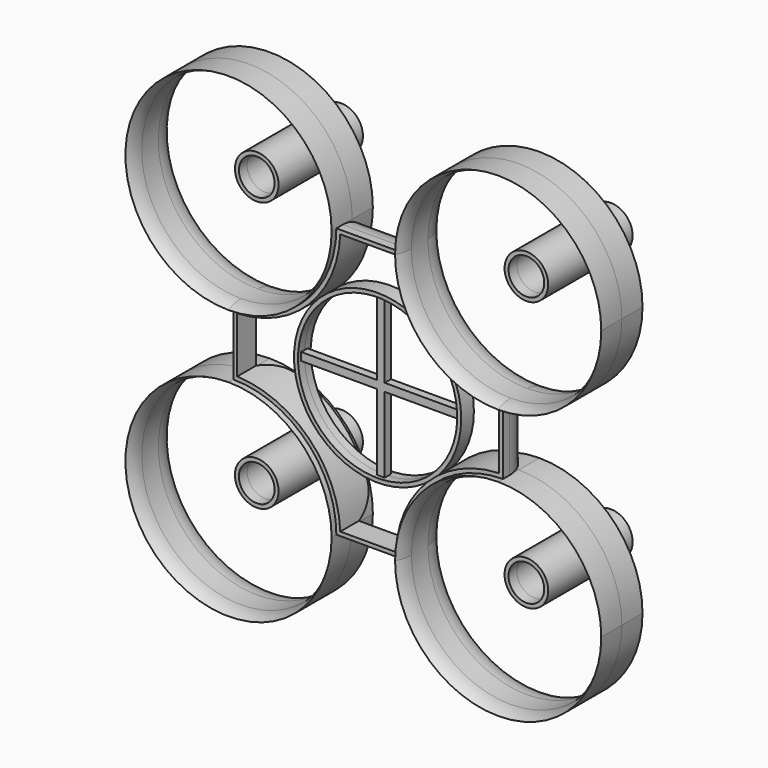
from build123d import *

# Parameters (mm, degrees)
F1_DEPTH       = 4.1275
F2_DEPTH       = 3.175
F3_R           = 15.875
F4_DEPTH       = 25.4
F6_DEPTH       = 25.4
F7_T2_ANGLE    = 270
F7_T4_ANGLE    = 90
F7_T6_ANGLE    = 270
F7_T8_ANGLE    = 90
F7_2_T2_ANGLE  = 90
F7_2_T4_ANGLE  = 270
F7_2_T6_ANGLE  = 90
F7_2_T8_ANGLE  = 270
F7_3_T2_ANGLE  = 90
F7_3_T4_ANGLE  = 89.999999553
F7_3_T6_ANGLE  = 180.000000447
F7_3_T8_ANGLE  = 90
F7_3_T10_ANGLE = 89.999999553
F7_3_T12_ANGLE = 180.000000447
F7_4_T2_ANGLE  = 180
F7_4_T4_ANGLE  = 89.999999553
F7_4_T6_ANGLE  = 90.000000447
F7_4_T8_ANGLE  = 180
F7_4_T10_ANGLE = 89.999999553
F7_4_T12_ANGLE = 90.000000447
F8_T1_DEPTH    = 35.56
F8_T3_DEPTH    = 35.56
F9_R           = 13.3878708116
F10_DEPTH      = 1.27
F11_DEPTH      = 0.635
F12_R          = 3.4925
F12_R_2        = 2.8575
F13_DEPTH      = 15.24
F13_DEPTH_BACK = 1.651


# Not quite as in the source:
# - a fillet or chamfer that OpenCascade refuses, or shapes differently, is made with other operations: its cross-section is extruded or revolved along the edge and cut away or added


with BuildPart() as f1:
    # F0 (on Front) → F1 (new body, symmetric)
    with BuildSketch(Plane.XZ):
        with BuildLine():
            ThreePointArc((-21.59, 5.08), (-9.9156670426, 9.9156670426), (-5.08, 21.59))
            ThreePointArc((-5.08, 21.59), (-33.2643329574, 33.2643329574), (-21.59, 5.08))
        make_face()
    extrude(amount=F1_DEPTH, both=True)


with BuildPart() as f1b:
    # F0 (on Front) → F1, piece 2 (new body, symmetric)
    with BuildSketch(Plane.XZ):
        with BuildLine():
            ThreePointArc((-5.08, -21.59), (-9.9156670426, -9.9156670426), (-21.59, -5.08))
            ThreePointArc((-21.59, -5.08), (-33.2643329574, -33.2643329574), (-5.08, -21.59))
        make_face()
    extrude(amount=F1_DEPTH, both=True)


with BuildPart() as f1c:
    # F0 (on Front) → F1, piece 3 (new body, symmetric)
    with BuildSketch(Plane.XZ):
        with BuildLine():
            ThreePointArc((38.1, -21.59), (33.2643329574, -9.9156670426), (21.59, -5.08))
            ThreePointArc((21.59, -5.08), (9.9156670426, -9.9156670426), (5.08, -21.59))
            ThreePointArc((5.08, -21.59), (21.59, -38.1), (38.1, -21.59))
        make_face()
    extrude(amount=F1_DEPTH, both=True)


with BuildPart() as f1d:
    # F0 (on Front) → F1, piece 4 (new body, symmetric)
    with BuildSketch(Plane.XZ):
        with BuildLine():
            ThreePointArc((38.1, 21.59), (21.59, 38.1), (5.08, 21.59))
            ThreePointArc((5.08, 21.59), (9.9156670426, 9.9156670426), (21.59, 5.08))
            ThreePointArc((21.59, 5.08), (33.2643329574, 9.9156670426), (38.1, 21.59))
        make_face()
    extrude(amount=F1_DEPTH, both=True)


with BuildPart() as f2:
    # F0 (on Front) → F2 (new body, symmetric)
    with BuildSketch(Plane.XZ):
        with BuildLine():
            Line((5.08, 21.59), (-5.08, 21.59))
            ThreePointArc((-5.08, 21.59), (-9.9156670426, 9.9156670426), (-21.59, 5.08))
            Line((-21.59, 5.08), (-21.59, -5.08))
            ThreePointArc((-21.59, -5.08), (-9.9156670426, -9.9156670426), (-5.08, -21.59))
            Line((-5.08, -21.59), (5.08, -21.59))
            ThreePointArc((5.08, -21.59), (9.9156670426, -9.9156670426), (21.59, -5.08))
            Line((21.59, -5.08), (21.59, 5.08))
            ThreePointArc((21.59, 5.08), (9.9156670426, 9.9156670426), (5.08, 21.59))
        make_face()
    extrude(amount=F2_DEPTH, both=True)

    # F5 (on face) → F6 (cut)
    with BuildSketch(Plane.XZ.offset(3.175)):
        with BuildLine():
            ThreePointArc((20.955, 4.4567632947), (9.4666542366, 9.4666542366), (4.4567632947, 20.955))
            Line((4.4567632947, 20.955), (-4.4567632947, 20.955))
            ThreePointArc((-4.4567632947, 20.955), (-9.4666542366, 9.4666542366), (-20.955, 4.4567632947))
            Line((-20.955, 4.4567632947), (-20.955, -4.4567632947))
            ThreePointArc((-20.955, -4.4567632947), (-9.4666542366, -9.4666542366), (-4.4567632947, -20.955))
            Line((-4.4567632947, -20.955), (4.4567632947, -20.955))
            ThreePointArc((4.4567632947, -20.955), (9.4666542366, -9.4666542366), (20.955, -4.4567632947))
            Line((20.955, -4.4567632947), (20.955, 4.4567632947))
        make_face()
    extrude(amount=-F6_DEPTH, mode=Mode.SUBTRACT)

    # F8: fillet of radius 5.08 on 4 edges, made by hand

    # F8_s2 → F8_t1 (cut)
    with BuildSketch(Plane.YZ.offset(-17.78)):
        with BuildLine():
            ThreePointArc((3.175, 16.51), (1.6871024484, 20.1021024484), (-1.905, 21.59))
            Line((-1.905, 21.59), (3.175, 21.59))
            Line((3.175, 21.59), (3.175, 16.51))
        make_face()
        with BuildLine():
            ThreePointArc((3.175, -16.51), (1.6871024484, -20.1021024484), (-1.905, -21.59))
            Line((-1.905, -21.59), (3.175, -21.59))
            Line((3.175, -21.59), (3.175, -16.51))
        make_face()
    extrude(amount=F8_T1_DEPTH, mode=Mode.SUBTRACT)

    # F8_s4 → F8_t3 (cut)
    with BuildSketch(Plane.XY.offset(-17.78)):
        with BuildLine():
            ThreePointArc((16.51, 3.175), (20.1021024484, 1.6871024484), (21.59, -1.905))
            Line((21.59, -1.905), (21.59, 3.175))
            Line((21.59, 3.175), (16.51, 3.175))
        make_face()
        with BuildLine():
            ThreePointArc((-16.51, 3.175), (-20.1021024484, 1.6871024484), (-21.59, -1.905))
            Line((-21.59, -1.905), (-21.59, 3.175))
            Line((-21.59, 3.175), (-16.51, 3.175))
        make_face()
    extrude(amount=F8_T3_DEPTH, mode=Mode.SUBTRACT)


with BuildPart() as f4_tool:
    # F3 (on face) → F4 (new body)
    with BuildSketch(Plane.XZ.offset(4.1275)):
        with Locations((-21.59, 21.59)):
            Circle(F3_R)
        with Locations((21.59, 21.59)):
            Circle(F3_R)
        with Locations((21.59, -21.59)):
            Circle(F3_R)
        with Locations((-21.59, -21.59)):
            Circle(F3_R)
    extrude(amount=-F4_DEPTH)


with BuildPart() as f1_1:
    add(f1.part)

    # F4: cut by f4_tool
    add(f4_tool.part, mode=Mode.SUBTRACT)

    # F7: fillet of radius 5.08 on 3 edges, made by hand

    # F7_s1 → F7_t2 (revolve, cut)
    with BuildSketch(Plane.XY.offset(21.59)):
        with BuildLine():
            ThreePointArc((-5.08, -4.1275), (-5.5536888497, -2.9381555752), (-5.715, -1.6681555752))
            Line((-5.715, -1.6681555752), (-5.715, -4.1275))
            Line((-5.715, -4.1275), (-5.08, -4.1275))
        make_face()
    revolve(axis=Axis((-21.59, -4.1275, 21.59), (0, -1, 0)), revolution_arc=F7_T2_ANGLE, mode=Mode.SUBTRACT)

    # F7_s3 → F7_t4 (revolve, cut)
    with BuildSketch(Plane.YZ.offset(-21.59)):
        with BuildLine():
            ThreePointArc((-4.1275, 5.08), (-2.9381555752, 5.5536888497), (-1.6681555752, 5.715))
            Line((-1.6681555752, 5.715), (-4.1275, 5.715))
            Line((-4.1275, 5.715), (-4.1275, 5.08))
        make_face()
    revolve(axis=Axis((-21.59, -4.1275, 21.59), (0, -1, 0)), revolution_arc=F7_T4_ANGLE, mode=Mode.SUBTRACT)

    # F7_s5 → F7_t6 (revolve, cut)
    with BuildSketch(Plane.XY.offset(21.59)):
        with BuildLine():
            ThreePointArc((-5.08, 4.1275), (-5.5536888497, 2.9381555752), (-5.715, 1.6681555752))
            Line((-5.715, 1.6681555752), (-5.715, 4.1275))
            Line((-5.715, 4.1275), (-5.08, 4.1275))
        make_face()
    revolve(axis=Axis((-21.59, 4.1275, 21.59), (0, -1, 0)), revolution_arc=F7_T6_ANGLE, mode=Mode.SUBTRACT)

    # F7_s7 → F7_t8 (revolve, cut)
    with BuildSketch(Plane.YZ.offset(-21.59)):
        with BuildLine():
            ThreePointArc((4.1275, 5.08), (2.9381555752, 5.5536888497), (1.6681555752, 5.715))
            Line((1.6681555752, 5.715), (4.1275, 5.715))
            Line((4.1275, 5.715), (4.1275, 5.08))
        make_face()
    revolve(axis=Axis((-21.59, 4.1275, 21.59), (0, -1, 0)), revolution_arc=F7_T8_ANGLE, mode=Mode.SUBTRACT)


with BuildPart() as f1b_1:
    add(f1b.part)

    # F4: cut by f4_tool
    add(f4_tool.part, mode=Mode.SUBTRACT)

    # F7#2: fillet of radius 5.08 on 3 edges, made by hand

    # F7_2_s1 → F7_2_t2 (revolve, cut)
    with BuildSketch(Plane.XY.offset(-21.59)):
        with BuildLine():
            ThreePointArc((-5.08, -4.1275), (-5.5536888497, -2.9381555752), (-5.715, -1.6681555752))
            Line((-5.715, -1.6681555752), (-5.715, -4.1275))
            Line((-5.715, -4.1275), (-5.08, -4.1275))
        make_face()
    revolve(axis=Axis((-21.59, -4.1275, -21.59), (0, -1, 0)), revolution_arc=F7_2_T2_ANGLE, mode=Mode.SUBTRACT)

    # F7_2_s3 → F7_2_t4 (revolve, cut)
    with BuildSketch(Plane.YZ.offset(-21.59)):
        with BuildLine():
            ThreePointArc((-4.1275, -5.08), (-2.9381555752, -5.5536888497), (-1.6681555752, -5.715))
            Line((-1.6681555752, -5.715), (-4.1275, -5.715))
            Line((-4.1275, -5.715), (-4.1275, -5.08))
        make_face()
    revolve(axis=Axis((-21.59, -4.1275, -21.59), (0, -1, 0)), revolution_arc=F7_2_T4_ANGLE, mode=Mode.SUBTRACT)

    # F7_2_s5 → F7_2_t6 (revolve, cut)
    with BuildSketch(Plane.XY.offset(-21.59)):
        with BuildLine():
            ThreePointArc((-5.08, 4.1275), (-5.5536888497, 2.9381555752), (-5.715, 1.6681555752))
            Line((-5.715, 1.6681555752), (-5.715, 4.1275))
            Line((-5.715, 4.1275), (-5.08, 4.1275))
        make_face()
    revolve(axis=Axis((-21.59, 4.1275, -21.59), (0, -1, 0)), revolution_arc=F7_2_T6_ANGLE, mode=Mode.SUBTRACT)

    # F7_2_s7 → F7_2_t8 (revolve, cut)
    with BuildSketch(Plane.YZ.offset(-21.59)):
        with BuildLine():
            ThreePointArc((4.1275, -5.08), (2.9381555752, -5.5536888497), (1.6681555752, -5.715))
            Line((1.6681555752, -5.715), (4.1275, -5.715))
            Line((4.1275, -5.715), (4.1275, -5.08))
        make_face()
    revolve(axis=Axis((-21.59, 4.1275, -21.59), (0, -1, 0)), revolution_arc=F7_2_T8_ANGLE, mode=Mode.SUBTRACT)


with BuildPart() as f1c_1:
    add(f1c.part)

    # F4: cut by f4_tool
    add(f4_tool.part, mode=Mode.SUBTRACT)

    # F7#3: fillet of radius 5.08 on 3 edges, made by hand

    # F7_3_s1 → F7_3_t2 (revolve, cut)
    with BuildSketch(Plane.XY.offset(-21.59)):
        with BuildLine():
            ThreePointArc((38.1, -4.1275), (37.6263111503, -2.9381555752), (37.465, -1.6681555752))
            Line((37.465, -1.6681555752), (37.465, -4.1275))
            Line((37.465, -4.1275), (38.1, -4.1275))
        make_face()
    revolve(axis=Axis((21.59, -4.1275, -21.59), (0, -1, 0)), revolution_arc=F7_3_T2_ANGLE, mode=Mode.SUBTRACT)

    # F7_3_s3 → F7_3_t4 (revolve, cut)
    with BuildSketch(Plane.YZ.offset(21.59)):
        with BuildLine():
            ThreePointArc((-4.1275, -5.08), (-2.9381555752, -5.5536888497), (-1.6681555752, -5.715))
            Line((-1.6681555752, -5.715), (-4.1275, -5.715))
            Line((-4.1275, -5.715), (-4.1275, -5.08))
        make_face()
    revolve(axis=Axis((21.59, -4.1275, -21.59), (0, -1, 0)), revolution_arc=F7_3_T4_ANGLE, mode=Mode.SUBTRACT)

    # F7_3_s5 → F7_3_t6 (revolve, cut)
    with BuildSketch(Plane.XY.offset(-21.59)):
        with BuildLine():
            ThreePointArc((5.08, -4.1275), (5.5536888497, -2.9381555752), (5.715, -1.6681555752))
            Line((5.715, -1.6681555752), (5.715, -4.1275))
            Line((5.715, -4.1275), (5.08, -4.1275))
        make_face()
    revolve(axis=Axis((21.59, -4.1275, -21.59), (0, -1, 0)), revolution_arc=F7_3_T6_ANGLE, mode=Mode.SUBTRACT)

    # F7_3_s7 → F7_3_t8 (revolve, cut)
    with BuildSketch(Plane.XY.offset(-21.59)):
        with BuildLine():
            ThreePointArc((38.1, 4.1275), (37.6263111503, 2.9381555752), (37.465, 1.6681555752))
            Line((37.465, 1.6681555752), (37.465, 4.1275))
            Line((37.465, 4.1275), (38.1, 4.1275))
        make_face()
    revolve(axis=Axis((21.59, 4.1275, -21.59), (0, -1, 0)), revolution_arc=F7_3_T8_ANGLE, mode=Mode.SUBTRACT)

    # F7_3_s9 → F7_3_t10 (revolve, cut)
    with BuildSketch(Plane.YZ.offset(21.59)):
        with BuildLine():
            ThreePointArc((4.1275, -5.08), (2.9381555752, -5.5536888497), (1.6681555752, -5.715))
            Line((1.6681555752, -5.715), (4.1275, -5.715))
            Line((4.1275, -5.715), (4.1275, -5.08))
        make_face()
    revolve(axis=Axis((21.59, 4.1275, -21.59), (0, -1, 0)), revolution_arc=F7_3_T10_ANGLE, mode=Mode.SUBTRACT)

    # F7_3_s11 → F7_3_t12 (revolve, cut)
    with BuildSketch(Plane.XY.offset(-21.59)):
        with BuildLine():
            ThreePointArc((5.08, 4.1275), (5.5536888497, 2.9381555752), (5.715, 1.6681555752))
            Line((5.715, 1.6681555752), (5.715, 4.1275))
            Line((5.715, 4.1275), (5.08, 4.1275))
        make_face()
    revolve(axis=Axis((21.59, 4.1275, -21.59), (0, -1, 0)), revolution_arc=F7_3_T12_ANGLE, mode=Mode.SUBTRACT)


with BuildPart() as f1d_1:
    add(f1d.part)

    # F4: cut by f4_tool
    add(f4_tool.part, mode=Mode.SUBTRACT)

    # F7#4: fillet of radius 5.08 on 3 edges, made by hand

    # F7_4_s1 → F7_4_t2 (revolve, cut)
    with BuildSketch(Plane.XY.offset(21.59)):
        with BuildLine():
            ThreePointArc((38.1, -4.1275), (37.6263111503, -2.9381555752), (37.465, -1.6681555752))
            Line((37.465, -1.6681555752), (37.465, -4.1275))
            Line((37.465, -4.1275), (38.1, -4.1275))
        make_face()
    revolve(axis=Axis((21.59, -4.1275, 21.59), (0, -1, 0)), revolution_arc=F7_4_T2_ANGLE, mode=Mode.SUBTRACT)

    # F7_4_s3 → F7_4_t4 (revolve, cut)
    with BuildSketch(Plane.XY.offset(21.59)):
        with BuildLine():
            ThreePointArc((5.08, -4.1275), (5.5536888497, -2.9381555752), (5.715, -1.6681555752))
            Line((5.715, -1.6681555752), (5.715, -4.1275))
            Line((5.715, -4.1275), (5.08, -4.1275))
        make_face()
    revolve(axis=Axis((21.59, -4.1275, 21.59), (0, -1, 0)), revolution_arc=F7_4_T4_ANGLE, mode=Mode.SUBTRACT)

    # F7_4_s5 → F7_4_t6 (revolve, cut)
    with BuildSketch(Plane.YZ.offset(21.59)):
        with BuildLine():
            ThreePointArc((-4.1275, 5.08), (-2.9381555752, 5.5536888497), (-1.6681555752, 5.715))
            Line((-1.6681555752, 5.715), (-4.1275, 5.715))
            Line((-4.1275, 5.715), (-4.1275, 5.08))
        make_face()
    revolve(axis=Axis((21.59, -4.1275, 21.59), (0, -1, 0)), revolution_arc=F7_4_T6_ANGLE, mode=Mode.SUBTRACT)

    # F7_4_s7 → F7_4_t8 (revolve, cut)
    with BuildSketch(Plane.XY.offset(21.59)):
        with BuildLine():
            ThreePointArc((38.1, 4.1275), (37.6263111503, 2.9381555752), (37.465, 1.6681555752))
            Line((37.465, 1.6681555752), (37.465, 4.1275))
            Line((37.465, 4.1275), (38.1, 4.1275))
        make_face()
    revolve(axis=Axis((21.59, 4.1275, 21.59), (0, -1, 0)), revolution_arc=F7_4_T8_ANGLE, mode=Mode.SUBTRACT)

    # F7_4_s9 → F7_4_t10 (revolve, cut)
    with BuildSketch(Plane.XY.offset(21.59)):
        with BuildLine():
            ThreePointArc((5.08, 4.1275), (5.5536888497, 2.9381555752), (5.715, 1.6681555752))
            Line((5.715, 1.6681555752), (5.715, 4.1275))
            Line((5.715, 4.1275), (5.08, 4.1275))
        make_face()
    revolve(axis=Axis((21.59, 4.1275, 21.59), (0, -1, 0)), revolution_arc=F7_4_T10_ANGLE, mode=Mode.SUBTRACT)

    # F7_4_s11 → F7_4_t12 (revolve, cut)
    with BuildSketch(Plane.YZ.offset(21.59)):
        with BuildLine():
            ThreePointArc((4.1275, 5.08), (2.9381555752, 5.5536888497), (1.6681555752, 5.715))
            Line((1.6681555752, 5.715), (4.1275, 5.715))
            Line((4.1275, 5.715), (4.1275, 5.08))
        make_face()
    revolve(axis=Axis((21.59, 4.1275, 21.59), (0, -1, 0)), revolution_arc=F7_4_T12_ANGLE, mode=Mode.SUBTRACT)


with BuildPart() as f10:
    # F9 (on Front) → F10 (new body, symmetric)
    with BuildSketch(Plane.XZ):
        Circle(F9_R)
        with BuildLine():
            ThreePointArc((12.7349784311, 0.635), (12.7468439941, 0.3175985367), (12.7508, 0))
            ThreePointArc((12.7508, 0), (12.7468439941, -0.3175985367), (12.7349784311, -0.635))
            ThreePointArc((12.7349784311, -0.635), (9.0161771456, -9.0161771456), (0.635, -12.7349784311))
            ThreePointArc((0.635, -12.7349784311), (0, -12.7508), (-0.635, -12.7349784311))
            ThreePointArc((-0.635, -12.7349784311), (-9.0161771456, -9.0161771456), (-12.7349784311, -0.635))
            ThreePointArc((-12.7349784311, -0.635), (-12.7508, 0), (-12.7349784311, 0.635))
            ThreePointArc((-12.7349784311, 0.635), (-9.0161771456, 9.0161771456), (-0.635, 12.7349784311))
            ThreePointArc((-0.635, 12.7349784311), (0, 12.7508), (0.635, 12.7349784311))
            ThreePointArc((0.635, 12.7349784311), (9.0161771456, 9.0161771456), (12.7349784311, 0.635))
        make_face(mode=Mode.SUBTRACT)
    extrude(amount=F10_DEPTH, both=True)

    # F9 (on Front) → F11 (join, symmetric)
    with BuildSketch(Plane.XZ):
        with BuildLine():
            ThreePointArc((12.7349784311, -0.635), (12.7468439941, -0.3175985367), (12.7508, 0))
            ThreePointArc((12.7508, 0), (12.7468439941, 0.3175985367), (12.7349784311, 0.635))
            Line((12.7349784311, 0.635), (0.635, 0.635))
            Line((0.635, 0.635), (0.635, 12.7349784311))
            ThreePointArc((0.635, 12.7349784311), (0, 12.7508), (-0.635, 12.7349784311))
            Line((-0.635, 12.7349784311), (-0.635, 0.635))
            Line((-0.635, 0.635), (-12.7349784311, 0.635))
            ThreePointArc((-12.7349784311, 0.635), (-12.7508, 0), (-12.7349784311, -0.635))
            Line((-12.7349784311, -0.635), (-0.635, -0.635))
            Line((-0.635, -0.635), (-0.635, -12.7349784311))
            ThreePointArc((-0.635, -12.7349784311), (0, -12.7508), (0.635, -12.7349784311))
            Line((0.635, -12.7349784311), (0.635, -0.635))
            Line((0.635, -0.635), (12.7349784311, -0.635))
        make_face()
    extrude(amount=F11_DEPTH, both=True)


with BuildPart() as f13:
    # F12 (on face) → F13 (new body, two sides)
    with BuildSketch(Plane(origin=(0, 3.175, 0), x_dir=(-1, 0, 0), z_dir=(0, 1, 0))) as f13_sk:
        with Locations((21.59, 21.59)):
            Circle(F12_R)
        with Locations((21.59, 21.59)):
            Circle(F12_R_2, mode=Mode.SUBTRACT)
    extrude(amount=F13_DEPTH)
    extrude(f13_sk.sketch, amount=-F13_DEPTH_BACK)


with BuildPart() as f13b:
    # F12 (on face) → F13, piece 2 (new body, two sides)
    with BuildSketch(Plane(origin=(0, 3.175, 0), x_dir=(-1, 0, 0), z_dir=(0, 1, 0))) as f13_2_sk:
        with Locations((-21.59, 21.59)):
            Circle(F12_R)
        with Locations((-21.59, 21.59)):
            Circle(F12_R_2, mode=Mode.SUBTRACT)
    extrude(amount=F13_DEPTH)
    extrude(f13_2_sk.sketch, amount=-F13_DEPTH_BACK)


with BuildPart() as f13c:
    # F12 (on face) → F13, piece 3 (new body, two sides)
    with BuildSketch(Plane(origin=(0, 3.175, 0), x_dir=(-1, 0, 0), z_dir=(0, 1, 0))) as f13_3_sk:
        with Locations((-21.59, -21.59)):
            Circle(F12_R)
        with Locations((-21.59, -21.59)):
            Circle(F12_R_2, mode=Mode.SUBTRACT)
    extrude(amount=F13_DEPTH)
    extrude(f13_3_sk.sketch, amount=-F13_DEPTH_BACK)


with BuildPart() as f13d:
    # F12 (on face) → F13, piece 4 (new body, two sides)
    with BuildSketch(Plane(origin=(0, 3.175, 0), x_dir=(-1, 0, 0), z_dir=(0, 1, 0))) as f13_4_sk:
        with Locations((21.59, -21.59)):
            Circle(F12_R)
        with Locations((21.59, -21.59)):
            Circle(F12_R_2, mode=Mode.SUBTRACT)
    extrude(amount=F13_DEPTH)
    extrude(f13_4_sk.sketch, amount=-F13_DEPTH_BACK)


solid = Compound([f2.part, f1_1.part, f1b_1.part, f1c_1.part, f1d_1.part, f10.part, f13.part, f13b.part, f13c.part, f13d.part])
